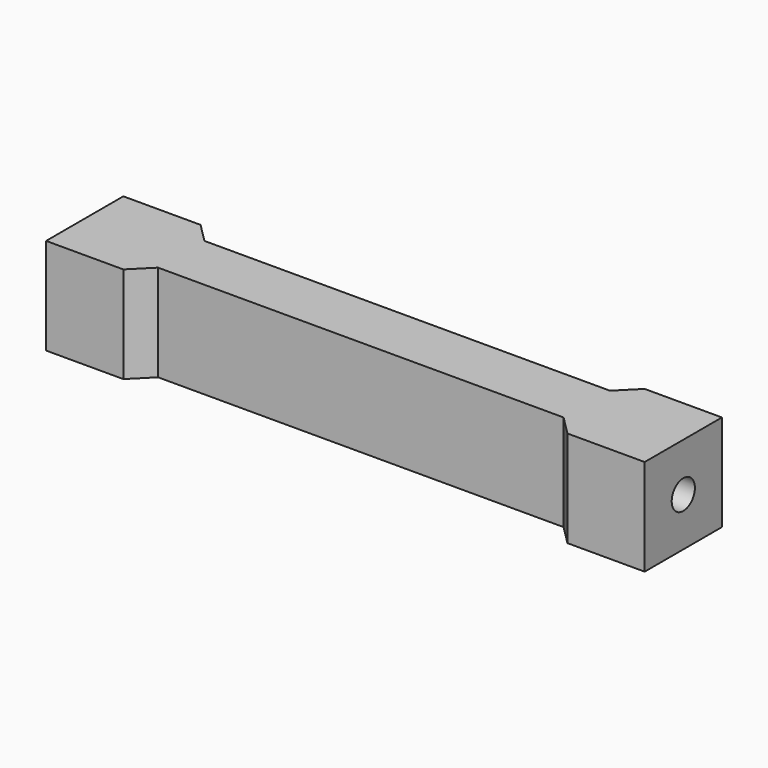
from build123d import *

# Parameters (mm, degrees)
F1_DEPTH = 10
F2_SIZE  = 1.99999
F3_R     = 1.5
F4_DEPTH = 15
F5_R     = 1.5
F6_DEPTH = 15


# Not quite as in the source:
# - a fillet or chamfer is up to 0.001 mm smaller than in the source, because OpenCascade refuses the exact size


with BuildPart() as f1:
    # F0 (on Top) → F1 (new body)
    with BuildSketch(Plane.XY):
        Polygon((-15.3143769915, 8.338528797), (-25.3143769915, 8.338528797), (-25.3143769915, -1.661471203), (-15.3143769915, -1.661471203), (-15.3143769915, 0.338528797), (26.6856230085, 0.338528797), (26.6856230085, -1.661471203), (36.6856230085, -1.661471203), (36.6856230085, 8.338528797), (26.6856230085, 8.338528797), (26.6856230085, 6.338528797), (-15.3143769915, 6.338528797), align=None)
    extrude(amount=F1_DEPTH)

    # F2 (size 2 in the source; OpenCascade refuses exactly that, so slightly less here)
    f2_edges = [f1.edges().sort_by_distance(p)[0] for p in [
        (-15.314377, 8.338529, 5),
        (26.685623, 8.338529, 5),
        (-15.314377, -1.661471, 5),
        (26.685623, -1.661471, 5),
    ]]
    chamfer(f2_edges, length=F2_SIZE)

    # F3 (on face) → F4 (cut)
    with BuildSketch(Plane.YZ.offset(36.6856230085)):
        with Locations((3.338528797, 5)):
            Circle(F3_R)
    extrude(amount=-F4_DEPTH, mode=Mode.SUBTRACT)

    # F5 (on face) → F6 (cut)
    with BuildSketch(Plane(origin=(-25.3143769915, 0, 0), x_dir=(0, -1, 0), z_dir=(-1, 0, 0))):
        with Locations((-3.338528797, 5)):
            Circle(F5_R)
    extrude(amount=-F6_DEPTH, mode=Mode.SUBTRACT)


solid = f1.part
